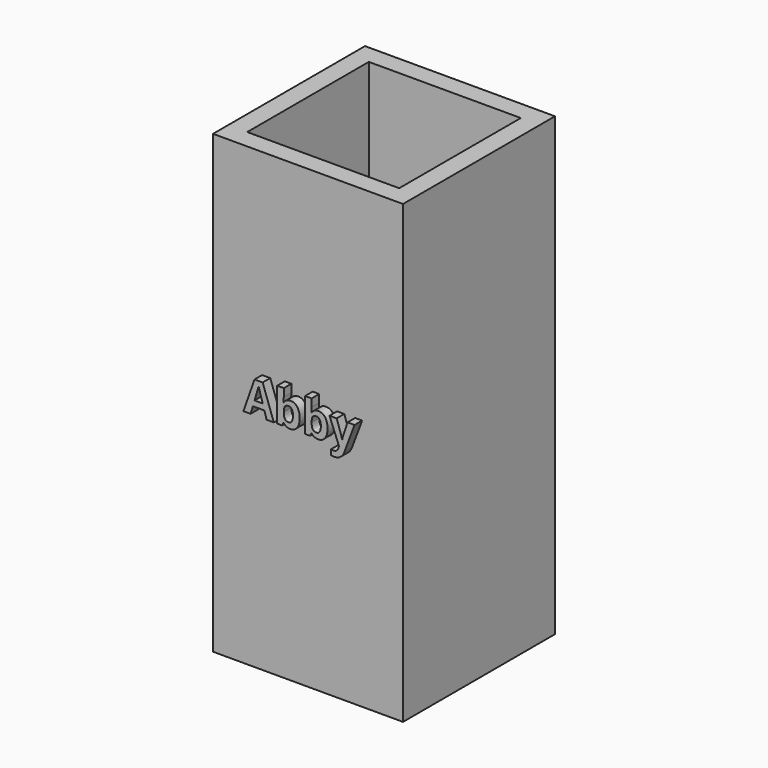
from build123d import *

# Parameters (mm, degrees)
F0_W         = 63.5
F0_H         = 152.4
F1_DEPTH     = 63.5
F2_W         = 50.8
F2_H         = 50.8
F3_DEPTH     = 139.7
F4_TEXT_SIZE = 14.7139753802
F5_DEPTH     = 3.175


# Not quite as in the source:
# - Text() gives the source's letters only with a copy of the font that has no kerning and outlines rounded to 1/6400 em; it was checked with that copy


with BuildPart() as f1:
    # F0 (on Front) → F1 (new body)
    with BuildSketch(Plane.XZ):
        with Locations((-1.0431338266, 49.3997552034)):
            Rectangle(F0_W, F0_H)
    extrude(amount=F1_DEPTH)

    # F2 (on face) → F3 (cut)
    with BuildSketch(Plane.XY.offset(125.5997552034)):
        with Locations((-1.0431338266, -31.75)):
            Rectangle(F2_W, F2_H)
    extrude(amount=-F3_DEPTH, mode=Mode.SUBTRACT)

    # F4 (on face) → F5 (join)
    with BuildSketch(Plane.XZ.offset(63.5)):
        with Locations((-20.0931338266, 49.3997552034)):
            Text('Abby', F4_TEXT_SIZE, font='Open Sans', font_style=FontStyle.BOLD, text_align=(TextAlign.LEFT, TextAlign.BOTTOM))
    extrude(amount=F5_DEPTH)


solid = f1.part
